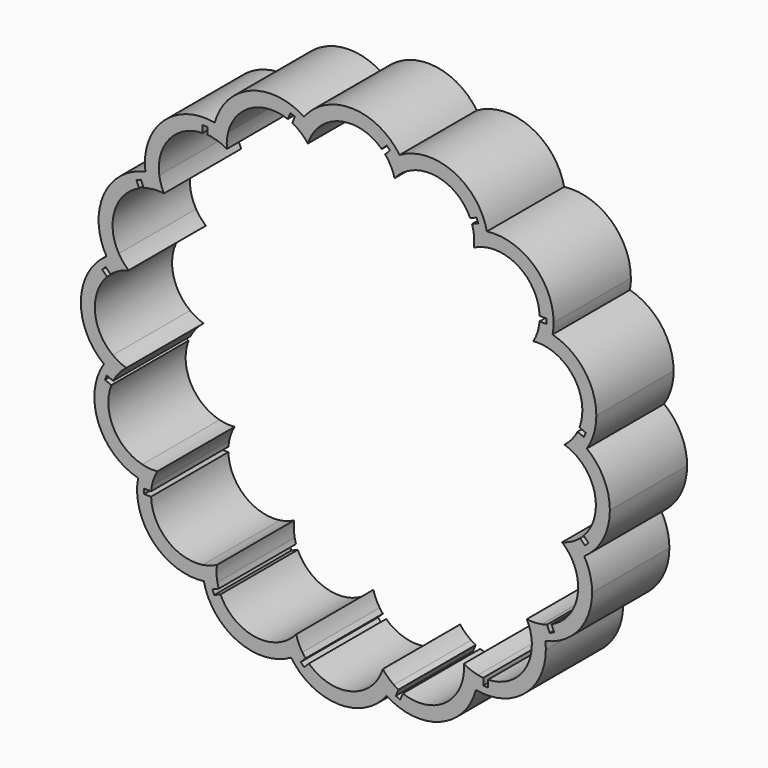
from build123d import *

# Parameters (mm, degrees)
F1_DEPTH = 14.52


with BuildPart() as f1:
    # F0 (on Front) → F1 (new body)
    with BuildSketch(Plane.XZ):
        with BuildLine():
            ThreePointArc((-19.9333001571, 29.0767800936), (-18.8383988511, 28.7630723121), (-17.8113981478, 28.2706385627))
            ThreePointArc((-17.8113981478, 28.2706385627), (-17.8122246799, 29.4095945579), (-17.6225246304, 30.5326419003))
            ThreePointArc((-17.6225246304, 30.5326419003), (-18.6077963784, 30.9046211349), (-19.6301585519, 31.1574146366))
            ThreePointArc((-19.6301585519, 31.1574146366), (-19.8434891082, 30.1260955579), (-19.9333001571, 29.0767800936))
        make_face()
        with BuildLine():
            ThreePointArc((-20.7306947559, 29.18563083), (-20.3303821446, 29.1430385555), (-19.9333001571, 29.0767800936))
            ThreePointArc((-19.9333001571, 29.0767800936), (-19.8434891082, 30.1260955579), (-19.6301585519, 31.1574146366))
            ThreePointArc((-19.6301585519, 31.1574146366), (-27.3602495357, 28.86978071), (-30.0593280828, 21.2735612162))
            ThreePointArc((-30.0593280828, 21.2735612162), (-29.018048711, 21.4312515397), (-27.9654260188, 21.4646347127))
            ThreePointArc((-27.9654260188, 21.4646347127), (-26.4406703088, 26.7876744669), (-21.4577037841, 29.2021468347))
            Line((-21.4577037841, 29.2021468347), (-21.4577037841, 30.2331540734))
            Line((-21.4577037841, 30.2331540734), (-20.7306947559, 30.2331540734))
            Line((-20.7306947559, 30.2331540734), (-20.7306947559, 29.18563083))
        make_face()
        with BuildLine():
            ThreePointArc((-19.6301585519, 31.1574146366), (-18.6077963784, 30.9046211349), (-17.6225246304, 30.5326419003))
            ThreePointArc((-17.6225246304, 30.5326419003), (-14.1767949141, 34.8669906313), (-8.6491555577, 35.1907735007))
            Line((-8.6491555577, 35.1907735007), (-8.2546061688, 36.1432999864))
            Line((-8.2546061688, 36.1432999864), (-7.5829374077, 35.8650856761))
            Line((-7.5829374077, 35.8650856761), (-7.983807198, 34.8973003918))
            ThreePointArc((-7.983807198, 34.8973003918), (-7.6302659276, 34.704757257), (-7.2887660222, 34.4915857222))
            ThreePointArc((-7.2887660222, 34.4915857222), (-6.8042357888, 35.4266576025), (-6.2124753293, 36.2978341212))
            ThreePointArc((-6.2124753293, 36.2978341212), (-14.2295877767, 37.1425137087), (-19.6301585519, 31.1574146366))
        make_face()
        with BuildLine():
            ThreePointArc((-6.2124753293, 36.2978341212), (-6.8042357888, 35.4266576025), (-7.2887660222, 34.4915857222))
            ThreePointArc((-7.2887660222, 34.4915857222), (-6.397259886, 33.7827569339), (-5.6368811938, 32.9347913176))
            ThreePointArc((-5.6368811938, 32.9347913176), (-5.2017852203, 33.98736575), (-4.5967536157, 34.9523311377))
            ThreePointArc((-4.5967536157, 34.9523311377), (-5.3646757273, 35.6730423134), (-6.2124753293, 36.2978341212))
        make_face()
        with BuildLine():
            ThreePointArc((-29.5431700389, 19.2352982773), (-28.4115623616, 19.3644706687), (-27.2742911945, 19.3025373607))
            ThreePointArc((-27.2742911945, 19.3025373607), (-27.7109144001, 20.3544791929), (-27.9654260188, 21.4646347127))
            ThreePointArc((-27.9654260188, 21.4646347127), (-29.018048711, 21.4312515397), (-30.0593280828, 21.2735612162))
            ThreePointArc((-30.0593280828, 21.2735612162), (-29.8617510925, 20.2391085584), (-29.5431700389, 19.2352982773))
        make_face()
        with BuildLine():
            ThreePointArc((-29.5431700389, 19.2352982773), (-29.8617510925, 20.2391085584), (-30.0593280828, 21.2735612162))
            ThreePointArc((-30.0593280828, 21.2735612162), (-36.3255613241, 16.2018853033), (-35.9122374016, 8.151000946))
            ThreePointArc((-35.9122374016, 8.151000946), (-35.0105661766, 8.6951681724), (-34.050844803, 9.1288314674))
            ThreePointArc((-34.050844803, 9.1288314674), (-34.6791933342, 14.6301776958), (-30.9995111239, 18.7677580311))
            Line((-30.9995111239, 18.7677580311), (-31.3940605128, 19.7202845169))
            Line((-31.3940605128, 19.7202845169), (-30.7223917517, 19.9984988271))
            Line((-30.7223917517, 19.9984988271), (-30.3215219615, 19.0307135427))
            ThreePointArc((-30.3215219615, 19.0307135427), (-29.9353819755, 19.1445564162), (-29.5431700389, 19.2352982773))
        make_face()
        with BuildLine():
            ThreePointArc((8.151000946, 35.9122374016), (1.0673997297, 39.760635693), (-6.2124753293, 36.2978341212))
            ThreePointArc((-6.2124753293, 36.2978341212), (-5.3646757273, 35.6730423134), (-4.5967536157, 34.9523311377))
            ThreePointArc((-4.5967536157, 34.9523311377), (0.2453689933, 37.6381235422), (5.4761481976, 35.8219239064))
            Line((5.4761481976, 35.8219239064), (6.2051804075, 36.5509561164))
            Line((6.2051804075, 36.5509561164), (6.7192534213, 36.0368831025))
            Line((6.7192534213, 36.0368831025), (5.9785426325, 35.2961723137))
            ThreePointArc((5.9785426325, 35.2961723137), (6.2314891084, 34.9829912655), (6.4654166667, 34.6553600917))
            ThreePointArc((6.4654166667, 34.6553600917), (7.2709007489, 35.3338321705), (8.151000946, 35.9122374016))
        make_face()
        with BuildLine():
            ThreePointArc((-34.050844803, 9.1288314674), (-35.0105661766, 8.6951681724), (-35.9122374016, 8.151000946))
            ThreePointArc((-35.9122374016, 8.151000946), (-35.3338321705, 7.2709007489), (-34.6553600917, 6.4654166667))
            ThreePointArc((-34.6553600917, 6.4654166667), (-33.659323054, 7.0178039054), (-32.5849206489, 7.3957998235))
            ThreePointArc((-32.5849206489, 7.3957998235), (-33.390868603, 8.2005788847), (-34.050844803, 9.1288314674))
        make_face()
        with BuildLine():
            ThreePointArc((-34.6553600917, 6.4654166667), (-35.3338321705, 7.2709007489), (-35.9122374016, 8.151000946))
            ThreePointArc((-35.9122374016, 8.151000946), (-39.760635693, 1.0673997297), (-36.2978341212, -6.2124753293))
            ThreePointArc((-36.2978341212, -6.2124753293), (-35.6730423134, -5.3646757273), (-34.9523311377, -4.5967536157))
            ThreePointArc((-34.9523311377, -4.5967536157), (-37.6381235422, 0.2453689933), (-35.8219239064, 5.4761481976))
            Line((-35.8219239064, 5.4761481976), (-36.5509561164, 6.2051804075))
            Line((-36.5509561164, 6.2051804075), (-36.0368831025, 6.7192534213))
            Line((-36.0368831025, 6.7192534213), (-35.2961723137, 5.9785426325))
            ThreePointArc((-35.2961723137, 5.9785426325), (-34.9829912655, 6.2314891084), (-34.6553600917, 6.4654166667))
        make_face()
        with BuildLine():
            ThreePointArc((9.1288314674, 34.050844803), (8.6951681724, 35.0105661766), (8.151000946, 35.9122374016))
            ThreePointArc((8.151000946, 35.9122374016), (7.2709007489, 35.3338321705), (6.4654166667, 34.6553600917))
            ThreePointArc((6.4654166667, 34.6553600917), (7.0178039054, 33.659323054), (7.3957998235, 32.5849206489))
            ThreePointArc((7.3957998235, 32.5849206489), (8.2005788847, 33.390868603), (9.1288314674, 34.050844803))
        make_face()
        with BuildLine():
            ThreePointArc((21.2735612162, 30.0593280828), (16.2018853033, 36.3255613241), (8.151000946, 35.9122374016))
            ThreePointArc((8.151000946, 35.9122374016), (8.6951681724, 35.0105661766), (9.1288314674, 34.050844803))
            ThreePointArc((9.1288314674, 34.050844803), (14.6301776958, 34.6791933342), (18.7677580311, 30.9995111239))
            Line((18.7677580311, 30.9995111239), (19.7202845169, 31.3940605128))
            Line((19.7202845169, 31.3940605128), (19.9984988271, 30.7223917517))
            Line((19.9984988271, 30.7223917517), (19.0307135427, 30.3215219615))
            ThreePointArc((19.0307135427, 30.3215219615), (19.1445564162, 29.9353819755), (19.2352982773, 29.5431700389))
            ThreePointArc((19.2352982773, 29.5431700389), (20.2391085584, 29.8617510925), (21.2735612162, 30.0593280828))
        make_face()
        with BuildLine():
            ThreePointArc((-34.9523311377, -4.5967536157), (-35.6730423134, -5.3646757273), (-36.2978341212, -6.2124753293))
            ThreePointArc((-36.2978341212, -6.2124753293), (-35.4266576025, -6.8042357888), (-34.4915857222, -7.2887660222))
            ThreePointArc((-34.4915857222, -7.2887660222), (-33.7827569339, -6.397259886), (-32.9347913176, -5.6368811938))
            ThreePointArc((-32.9347913176, -5.6368811938), (-33.98736575, -5.2017852203), (-34.9523311377, -4.5967536157))
        make_face()
        with BuildLine():
            ThreePointArc((-34.4915857222, -7.2887660222), (-35.4266576025, -6.8042357888), (-36.2978341212, -6.2124753293))
            ThreePointArc((-36.2978341212, -6.2124753293), (-37.1425137087, -14.2295877767), (-31.1574146366, -19.6301585519))
            ThreePointArc((-31.1574146366, -19.6301585519), (-30.9046211349, -18.6077963784), (-30.5326419003, -17.6225246304))
            ThreePointArc((-30.5326419003, -17.6225246304), (-34.8669906313, -14.1767949141), (-35.1907735007, -8.6491555577))
            Line((-35.1907735007, -8.6491555577), (-36.1432999864, -8.2546061688))
            Line((-36.1432999864, -8.2546061688), (-35.8650856761, -7.5829374077))
            Line((-35.8650856761, -7.5829374077), (-34.8973003918, -7.983807198))
            ThreePointArc((-34.8973003918, -7.983807198), (-34.704757257, -7.6302659276), (-34.4915857222, -7.2887660222))
        make_face()
        with BuildLine():
            ThreePointArc((21.4680171211, 28.2105745581), (21.4192694259, 29.140050579), (21.2735612162, 30.0593280828))
            ThreePointArc((21.2735612162, 30.0593280828), (20.2391085584, 29.8617510925), (19.2352982773, 29.5431700389))
            ThreePointArc((19.2352982773, 29.5431700389), (19.3343298848, 28.880140521), (19.3674481899, 28.2105745581))
            ThreePointArc((19.3674481899, 28.2105745581), (19.3512010302, 27.7413091874), (19.3025373607, 27.2742911945))
            ThreePointArc((19.3025373607, 27.2742911945), (20.3544791929, 27.7109144001), (21.4646347127, 27.9654260188))
            ThreePointArc((21.4646347127, 27.9654260188), (21.4671714788, 28.0879886219), (21.4680171211, 28.2105745581))
        make_face()
        with BuildLine():
            ThreePointArc((31.3059547836, 21.2480779737), (28.2839660674, 27.9242866504), (21.2735612162, 30.0593280828))
            ThreePointArc((21.2735612162, 30.0593280828), (21.4192694259, 29.140050579), (21.4680171211, 28.2105745581))
            ThreePointArc((21.4680171211, 28.2105745581), (21.4671714788, 28.0879886219), (21.4646347127, 27.9654260188))
            ThreePointArc((21.4646347127, 27.9654260188), (26.7876744669, 26.4406703088), (29.2021468347, 21.4577037841))
            Line((29.2021468347, 21.4577037841), (30.2331540734, 21.4577037841))
            Line((30.2331540734, 21.4577037841), (30.2331540734, 20.7306947559))
            Line((30.2331540734, 20.7306947559), (29.18563083, 20.7306947559))
            ThreePointArc((29.18563083, 20.7306947559), (29.1430385555, 20.3303821446), (29.0767800936, 19.9333001571))
            ThreePointArc((29.0767800936, 19.9333001571), (30.1260955579, 19.8434891082), (31.1574146366, 19.6301585519))
            ThreePointArc((31.1574146366, 19.6301585519), (31.2687418225, 20.435716073), (31.3059547836, 21.2480779737))
        make_face()
        with BuildLine():
            ThreePointArc((-30.5326419003, -17.6225246304), (-30.9046211349, -18.6077963784), (-31.1574146366, -19.6301585519))
            ThreePointArc((-31.1574146366, -19.6301585519), (-30.1260955579, -19.8434891082), (-29.0767800936, -19.9333001571))
            ThreePointArc((-29.0767800936, -19.9333001571), (-28.7630723121, -18.8383988511), (-28.2706385627, -17.8113981478))
            ThreePointArc((-28.2706385627, -17.8113981478), (-29.4095945579, -17.8122246799), (-30.5326419003, -17.6225246304))
        make_face()
        with BuildLine():
            ThreePointArc((-29.0767800936, -19.9333001571), (-30.1260955579, -19.8434891082), (-31.1574146366, -19.6301585519))
            ThreePointArc((-31.1574146366, -19.6301585519), (-28.86978071, -27.3602495357), (-21.2735612162, -30.0593280828))
            ThreePointArc((-21.2735612162, -30.0593280828), (-21.4312515397, -29.018048711), (-21.4646347127, -27.9654260188))
            ThreePointArc((-21.4646347127, -27.9654260188), (-26.7876744669, -26.4406703088), (-29.2021468347, -21.4577037841))
            Line((-29.2021468347, -21.4577037841), (-30.2331540734, -21.4577037841))
            Line((-30.2331540734, -21.4577037841), (-30.2331540734, -20.7306947559))
            Line((-30.2331540734, -20.7306947559), (-29.18563083, -20.7306947559))
            ThreePointArc((-29.18563083, -20.7306947559), (-29.1430385555, -20.3303821446), (-29.0767800936, -19.9333001571))
        make_face()
        with BuildLine():
            ThreePointArc((31.1574146366, 19.6301585519), (30.1260955579, 19.8434891082), (29.0767800936, 19.9333001571))
            ThreePointArc((29.0767800936, 19.9333001571), (28.7630723121, 18.8383988511), (28.2706385627, 17.8113981478))
            ThreePointArc((28.2706385627, 17.8113981478), (29.4095945579, 17.8122246799), (30.5326419003, 17.6225246304))
            ThreePointArc((30.5326419003, 17.6225246304), (30.9046211349, 18.6077963784), (31.1574146366, 19.6301585519))
        make_face()
        with BuildLine():
            ThreePointArc((31.1574146366, 19.6301585519), (30.9046211349, 18.6077963784), (30.5326419003, 17.6225246304))
            ThreePointArc((30.5326419003, 17.6225246304), (34.2063063999, 15.2092232514), (35.6300230102, 11.0507541322))
            ThreePointArc((35.6300230102, 11.0507541322), (35.5193073194, 9.8300355073), (35.1907735007, 8.6491555577))
            Line((35.1907735007, 8.6491555577), (36.1432999864, 8.2546061688))
            Line((36.1432999864, 8.2546061688), (35.8650856761, 7.5829374077))
            Line((35.8650856761, 7.5829374077), (34.8973003918, 7.983807198))
            ThreePointArc((34.8973003918, 7.983807198), (34.704757257, 7.6302659276), (34.4915857222, 7.2887660222))
            ThreePointArc((34.4915857222, 7.2887660222), (35.4266576025, 6.8042357888), (36.2978341212, 6.2124753293))
            ThreePointArc((36.2978341212, 6.2124753293), (37.3648763566, 8.5277729221), (37.7305919414, 11.0507541322))
            ThreePointArc((37.7305919414, 11.0507541322), (35.8983998761, 16.4547535788), (31.1574146366, 19.6301585519))
        make_face()
        with BuildLine():
            ThreePointArc((-21.4646347127, -27.9654260188), (-21.4312515397, -29.018048711), (-21.2735612162, -30.0593280828))
            ThreePointArc((-21.2735612162, -30.0593280828), (-20.2391085584, -29.8617510925), (-19.2352982773, -29.5431700389))
            ThreePointArc((-19.2352982773, -29.5431700389), (-19.3644706687, -28.4115623616), (-19.3025373607, -27.2742911945))
            ThreePointArc((-19.3025373607, -27.2742911945), (-20.3544791929, -27.7109144001), (-21.4646347127, -27.9654260188))
        make_face()
        with BuildLine():
            ThreePointArc((-19.2352982773, -29.5431700389), (-20.2391085584, -29.8617510925), (-21.2735612162, -30.0593280828))
            ThreePointArc((-21.2735612162, -30.0593280828), (-16.2018853033, -36.3255613241), (-8.151000946, -35.9122374016))
            ThreePointArc((-8.151000946, -35.9122374016), (-8.6951681724, -35.0105661766), (-9.1288314674, -34.050844803))
            ThreePointArc((-9.1288314674, -34.050844803), (-14.6301776958, -34.6791933342), (-18.7677580311, -30.9995111239))
            Line((-18.7677580311, -30.9995111239), (-19.7202845169, -31.3940605128))
            Line((-19.7202845169, -31.3940605128), (-19.9984988271, -30.7223917517))
            Line((-19.9984988271, -30.7223917517), (-19.0307135427, -30.3215219615))
            ThreePointArc((-19.0307135427, -30.3215219615), (-19.1445564162, -29.9353819755), (-19.2352982773, -29.5431700389))
        make_face()
        with BuildLine():
            ThreePointArc((36.2978341212, 6.2124753293), (35.4266576025, 6.8042357888), (34.4915857222, 7.2887660222))
            ThreePointArc((34.4915857222, 7.2887660222), (33.7827569339, 6.397259886), (32.9347913176, 5.6368811938))
            ThreePointArc((32.9347913176, 5.6368811938), (33.98736575, 5.2017852203), (34.9523311377, 4.5967536157))
            ThreePointArc((34.9523311377, 4.5967536157), (35.6730423134, 5.3646757273), (36.2978341212, 6.2124753293))
        make_face()
        with BuildLine():
            ThreePointArc((36.2978341212, 6.2124753293), (35.6730423134, 5.3646757273), (34.9523311377, 4.5967536157))
            ThreePointArc((34.9523311377, 4.5967536157), (36.9478118077, 2.2036839475), (37.6632668955, -0.8289468507))
            ThreePointArc((37.6632668955, -0.8289468507), (37.1861563135, -3.3282979846), (35.8219239064, -5.4761481976))
            Line((35.8219239064, -5.4761481976), (36.5509561164, -6.2051804075))
            Line((36.5509561164, -6.2051804075), (36.0368831025, -6.7192534213))
            Line((36.0368831025, -6.7192534213), (35.2961723137, -5.9785426325))
            ThreePointArc((35.2961723137, -5.9785426325), (34.9829912655, -6.2314891084), (34.6553600917, -6.4654166667))
            ThreePointArc((34.6553600917, -6.4654166667), (35.3338321705, -7.2709007489), (35.9122374016, -8.151000946))
            ThreePointArc((35.9122374016, -8.151000946), (38.7422044321, -4.9655906172), (39.7638358267, -0.8289468507))
            ThreePointArc((39.7638358267, -0.8289468507), (38.8503830948, 3.0951706978), (36.2978341212, 6.2124753293))
        make_face()
        with BuildLine():
            ThreePointArc((-9.1288314674, -34.050844803), (-8.6951681724, -35.0105661766), (-8.151000946, -35.9122374016))
            ThreePointArc((-8.151000946, -35.9122374016), (-7.2709007489, -35.3338321705), (-6.4654166667, -34.6553600917))
            ThreePointArc((-6.4654166667, -34.6553600917), (-7.0178039054, -33.659323054), (-7.3957998235, -32.5849206489))
            ThreePointArc((-7.3957998235, -32.5849206489), (-8.2005788847, -33.390868603), (-9.1288314674, -34.050844803))
        make_face()
        with BuildLine():
            ThreePointArc((-6.4654166667, -34.6553600917), (-7.2709007489, -35.3338321705), (-8.151000946, -35.9122374016))
            ThreePointArc((-8.151000946, -35.9122374016), (-1.0673997297, -39.760635693), (6.2124753293, -36.2978341212))
            ThreePointArc((6.2124753293, -36.2978341212), (5.3646757273, -35.6730423134), (4.5967536157, -34.9523311377))
            ThreePointArc((4.5967536157, -34.9523311377), (-0.2453689933, -37.6381235422), (-5.4761481976, -35.8219239064))
            Line((-5.4761481976, -35.8219239064), (-6.2051804075, -36.5509561164))
            Line((-6.2051804075, -36.5509561164), (-6.7192534213, -36.0368831025))
            Line((-6.7192534213, -36.0368831025), (-5.9785426325, -35.2961723137))
            ThreePointArc((-5.9785426325, -35.2961723137), (-6.2314891084, -34.9829912655), (-6.4654166667, -34.6553600917))
        make_face()
        with BuildLine():
            ThreePointArc((35.9122374016, -8.151000946), (35.3338321705, -7.2709007489), (34.6553600917, -6.4654166667))
            ThreePointArc((34.6553600917, -6.4654166667), (33.659323054, -7.0178039054), (32.5849206489, -7.3957998235))
            ThreePointArc((32.5849206489, -7.3957998235), (33.390868603, -8.2005788847), (34.050844803, -9.1288314674))
            ThreePointArc((34.050844803, -9.1288314674), (35.0105661766, -8.6951681724), (35.9122374016, -8.151000946))
        make_face()
        with BuildLine():
            ThreePointArc((35.9122374016, -8.151000946), (35.0105661766, -8.6951681724), (34.050844803, -9.1288314674))
            ThreePointArc((34.050844803, -9.1288314674), (34.7551317857, -10.7921980136), (34.9955745581, -12.5824481899))
            ThreePointArc((34.9955745581, -12.5824481899), (33.9096604321, -16.2643831704), (30.9995111239, -18.7677580311))
            Line((30.9995111239, -18.7677580311), (31.3940605128, -19.7202845169))
            Line((31.3940605128, -19.7202845169), (30.7223917517, -19.9984988271))
            Line((30.7223917517, -19.9984988271), (30.3215219615, -19.0307135427))
            ThreePointArc((30.3215219615, -19.0307135427), (29.9353819755, -19.1445564162), (29.5431700389, -19.2352982773))
            ThreePointArc((29.5431700389, -19.2352982773), (29.8617510925, -20.2391085584), (30.0593280828, -21.2735612162))
            ThreePointArc((30.0593280828, -21.2735612162), (35.1163895756, -18.1737856127), (37.0961434893, -12.5824481899))
            ThreePointArc((37.0961434893, -12.5824481899), (36.7950661363, -10.2890141763), (35.9122374016, -8.151000946))
        make_face()
        with BuildLine():
            ThreePointArc((4.5967536157, -34.9523311377), (5.3646757273, -35.6730423134), (6.2124753293, -36.2978341212))
            ThreePointArc((6.2124753293, -36.2978341212), (6.8042357888, -35.4266576025), (7.2887660222, -34.4915857222))
            ThreePointArc((7.2887660222, -34.4915857222), (6.397259886, -33.7827569339), (5.6368811938, -32.9347913176))
            ThreePointArc((5.6368811938, -32.9347913176), (5.2017852203, -33.98736575), (4.5967536157, -34.9523311377))
        make_face()
        with BuildLine():
            ThreePointArc((7.2887660222, -34.4915857222), (6.8042357888, -35.4266576025), (6.2124753293, -36.2978341212))
            ThreePointArc((6.2124753293, -36.2978341212), (14.2295877767, -37.1425137087), (19.6301585519, -31.1574146366))
            ThreePointArc((19.6301585519, -31.1574146366), (18.6077963784, -30.9046211349), (17.6225246304, -30.5326419003))
            ThreePointArc((17.6225246304, -30.5326419003), (14.1767949141, -34.8669906313), (8.6491555577, -35.1907735007))
            Line((8.6491555577, -35.1907735007), (8.2546061688, -36.1432999864))
            Line((8.2546061688, -36.1432999864), (7.5829374077, -35.8650856761))
            Line((7.5829374077, -35.8650856761), (7.983807198, -34.8973003918))
            ThreePointArc((7.983807198, -34.8973003918), (7.6302659276, -34.704757257), (7.2887660222, -34.4915857222))
        make_face()
        with BuildLine():
            ThreePointArc((30.0593280828, -21.2735612162), (29.8617510925, -20.2391085584), (29.5431700389, -19.2352982773))
            ThreePointArc((29.5431700389, -19.2352982773), (28.4115623616, -19.3644706687), (27.2742911945, -19.3025373607))
            ThreePointArc((27.2742911945, -19.3025373607), (27.7109144001, -20.3544791929), (27.9654260188, -21.4646347127))
            ThreePointArc((27.9654260188, -21.4646347127), (29.018048711, -21.4312515397), (30.0593280828, -21.2735612162))
        make_face()
        with BuildLine():
            ThreePointArc((30.0593280828, -21.2735612162), (29.018048711, -21.4312515397), (27.9654260188, -21.4646347127))
            ThreePointArc((27.9654260188, -21.4646347127), (28.0161438528, -21.9413146082), (28.0330779737, -22.4203858525))
            ThreePointArc((28.0330779737, -22.4203858525), (26.1193476298, -27.1434099831), (21.4577037841, -29.2021468347))
            Line((21.4577037841, -29.2021468347), (21.4577037841, -30.2331540734))
            Line((21.4577037841, -30.2331540734), (20.7306947559, -30.2331540734))
            Line((20.7306947559, -30.2331540734), (20.7306947559, -29.18563083))
            ThreePointArc((20.7306947559, -29.18563083), (20.3303821446, -29.1430385555), (19.9333001571, -29.0767800936))
            ThreePointArc((19.9333001571, -29.0767800936), (19.8434891082, -30.1260955579), (19.6301585519, -31.1574146366))
            ThreePointArc((19.6301585519, -31.1574146366), (26.9303838737, -29.25154497), (30.1336469049, -22.4203858525))
            ThreePointArc((30.1336469049, -22.4203858525), (30.1150477336, -21.8457707566), (30.0593280828, -21.2735612162))
        make_face()
        with BuildLine():
            ThreePointArc((17.6225246304, -30.5326419003), (18.6077963784, -30.9046211349), (19.6301585519, -31.1574146366))
            ThreePointArc((19.6301585519, -31.1574146366), (19.8434891082, -30.1260955579), (19.9333001571, -29.0767800936))
            ThreePointArc((19.9333001571, -29.0767800936), (18.8383988511, -28.7630723121), (17.8113981478, -28.2706385627))
            ThreePointArc((17.8113981478, -28.2706385627), (17.8296624014, -28.5575727069), (17.8357541322, -28.8450230102))
            ThreePointArc((17.8357541322, -28.8450230102), (17.7822356864, -29.6955411374), (17.6225246304, -30.5326419003))
        make_face()
    extrude(amount=F1_DEPTH)


solid = f1.part
